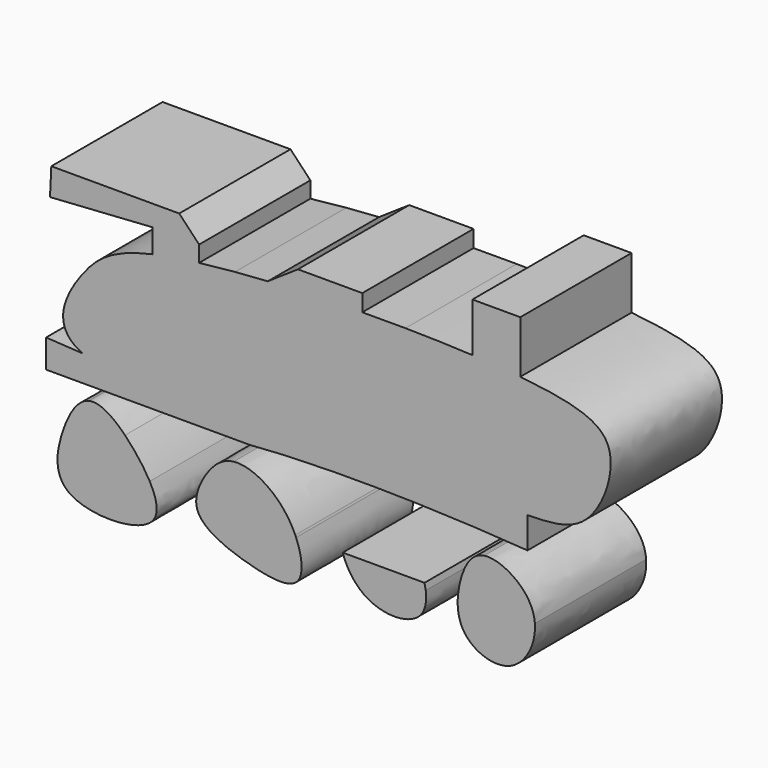
from build123d import *

# Parameters (mm, degrees)
F1_DEPTH = 25.4


with BuildPart() as f1:
    # F0 (on Front) → F1 (new body)
    with BuildSketch(Plane.XZ):
        with BuildLine():
            add(Edge.make_bspline(
                [(0, 6.2092236012), (0.399712228, 6.2271987583), (0.8012564022, 6.2442227103), (1.204486331, 6.2603151334)],
                knots=[0.5892572468, 0.5892572468, 0.5892572468, 0.5892572468, 0.5931096409, 0.5931096409, 0.5931096409, 0.5931096409], degree=3))
            add(Edge.make_bspline(
                [(1.204486331, 6.2603151334), (8.6074057831, 6.5557567752), (16.5785169504, 6.5372221525), (24.2131851795, 6.3264688191)],
                knots=[0.5931096409, 0.5931096409, 0.5931096409, 0.5931096409, 0.6638359458, 0.6638359458, 0.6638359458, 0.6638359458], degree=3))
            add(Edge.make_bspline(
                [(24.2131851795, 6.3264688191), (31.3805995307, 6.1286139261), (38.2514924404, 5.7613485246), (44.0773665905, 5.3254151655)],
                knots=[0.6638359458, 0.6638359458, 0.6638359458, 0.6638359458, 0.7302336879, 0.7302336879, 0.7302336879, 0.7302336879], degree=3))
            Line((44.0773665905, 5.3254151655), (44.0773665905, 10.5862493981))
            Line((44.0773665905, 10.5862493981), (-6.6354808577, 10.5862493981))
            Line((-6.6354808577, 10.5862493981), (-6.6354808577, 5.8050151421))
            add(Edge.make_bspline(
                [(-6.6354808577, 5.8050151421), (-4.875055728, 5.9437108093), (-3.0555777464, 6.0588505348), (-1.1922870019, 6.1524855288)],
                knots=[0.5672778823, 0.5672778823, 0.5672778823, 0.5672778823, 0.5854087698, 0.5854087698, 0.5854087698, 0.5854087698], degree=3))
            add(Edge.make_bspline(
                [(-1.1922870019, 6.1524855288), (-0.5897237764, 6.2718706989), (-0.1594076167, 6.2963081791), (0, 6.2092236012)],
                knots=[0.9136960461, 0.9136960461, 0.9136960461, 0.9136960461, 0.9595308359, 0.9595308359, 0.9595308359, 0.9595308359], degree=3))
        make_face()
        with BuildLine():
            add(Edge.make_bspline(
                [(-1.1922870019, 6.1524855288), (-0.7967833881, 6.172360569), (-0.3993058054, 6.191266721), (0, 6.2092236012)],
                knots=[0.5854087698, 0.5854087698, 0.5854087698, 0.5854087698, 0.5892572468, 0.5892572468, 0.5892572468, 0.5892572468], degree=3))
            add(Edge.make_bspline(
                [(-1.1922870019, 6.1524855288), (-0.5897237764, 6.2718706989), (-0.1594076167, 6.2963081791), (0, 6.2092236012)],
                knots=[0.9136960461, 0.9136960461, 0.9136960461, 0.9136960461, 0.9595308359, 0.9595308359, 0.9595308359, 0.9595308359], degree=3))
        make_face()
        with BuildLine():
            Line((-6.6354808577, 10.5862493981), (44.0773665905, 10.5862493981))
            Line((44.0773665905, 10.5862493981), (44.0773665905, 11.0193416477))
            add(Edge.make_bspline(
                [(42.7648406655, 32.815128364), (44.8295052016, 32.6085821778), (54.6822830844, 31.3655556574), (61.7602511034, 27.526332345), (55.8924998888, 11.2180255433), (47.9060181569, 11.0837244515), (44.0773665905, 11.0193416477)],
                knots=[0.6661346609, 0.6661346609, 0.6661346609, 0.6661346609, 0.6910717984, 0.7961772676, 0.9022891118, 1, 1, 1, 1], degree=3))
            add(Edge.make_bspline(
                [(34.0162292123, 33.4549068765), (37.1606205037, 33.2940351137), (40.1078698163, 33.0809280549), (42.7648406655, 32.815128364)],
                knots=[0.6340436135, 0.6340436135, 0.6340436135, 0.6340436135, 0.6661346609, 0.6661346609, 0.6661346609, 0.6661346609], degree=3))
            add(Edge.make_bspline(
                [(21.7825102865, 33.8114244437), (26.0413693418, 33.7699485679), (30.1758364775, 33.6513871144), (34.0162292123, 33.4549068765)],
                knots=[0.5948493104, 0.5948493104, 0.5948493104, 0.5948493104, 0.6340436135, 0.6340436135, 0.6340436135, 0.6340436135], degree=3))
            add(Edge.make_bspline(
                [(13.9097691545, 33.8017193911), (16.5545841031, 33.8333593914), (19.1915664693, 33.8366569444), (21.7825102865, 33.8114244437)],
                knots=[0.5710048404, 0.5710048404, 0.5710048404, 0.5710048404, 0.5948493104, 0.5948493104, 0.5948493104, 0.5948493104], degree=3))
            add(Edge.make_bspline(
                [(-3.3457321455, 33.1775619897), (2.1686140885, 33.5229891451), (8.058360875, 33.7317188187), (13.9097691545, 33.8017193911)],
                knots=[0.5182511573, 0.5182511573, 0.5182511573, 0.5182511573, 0.5710048404, 0.5710048404, 0.5710048404, 0.5710048404], degree=3))
            add(Edge.make_bspline(
                [(-9.333324452, 32.734493452), (-7.4038813376, 32.9010999132), (-5.4008780095, 33.0488244822), (-3.3457321455, 33.1775619897)],
                knots=[0.4985903473, 0.4985903473, 0.4985903473, 0.4985903473, 0.5182511573, 0.5182511573, 0.5182511573, 0.5182511573], degree=3))
            add(Edge.make_bspline(
                [(-15.8928215503, 32.0572180032), (-13.8354654472, 32.3097697763), (-11.6368180938, 32.5355879122), (-9.333324452, 32.734493452)],
                knots=[0.4751180042, 0.4751180042, 0.4751180042, 0.4751180042, 0.4985903473, 0.4985903473, 0.4985903473, 0.4985903473], degree=3))
            add(Edge.make_bspline(
                [(-19.5242251205, 31.5602992608), (-18.373006051, 31.7360479999), (-17.1597016187, 31.9017015094), (-15.8928215503, 32.0572180032)],
                knots=[0.4606641896, 0.4606641896, 0.4606641896, 0.4606641896, 0.4751180042, 0.4751180042, 0.4751180042, 0.4751180042], degree=3))
            add(Edge.make_bspline(
                [(-24.4341921061, 30.662516132), (-22.9708218581, 30.986326574), (-21.3233394805, 31.2856407804), (-19.5242251205, 31.5602992608)],
                knots=[0.4380759038, 0.4380759038, 0.4380759038, 0.4380759038, 0.4606641896, 0.4606641896, 0.4606641896, 0.4606641896], degree=3))
            add(Edge.make_bspline(
                [(-37.1303893626, 10.5862493981), (-39.6437434771, 11.654431227), (-42.1487635772, 15.6052377938), (-36.5862269371, 25.0979771624), (-31.6870538917, 29.0576233278), (-24.4341921061, 30.662516132)],
                knots=[0.1637001806, 0.1637001806, 0.1637001806, 0.1637001806, 0.2371830276, 0.326122203, 0.4380759038, 0.4380759038, 0.4380759038, 0.4380759038], degree=3))
            add(Edge.make_bspline(
                [(-6.6354808577, 10.5862493981), (-19.0833938627, 9.3964373169), (-31.5313068676, 8.2066252357), (-37.1303893626, 10.5862493981)],
                knots=[0, 0, 0, 0, 0.1637001806, 0.1637001806, 0.1637001806, 0.1637001806], degree=3))
        make_face()
        with BuildLine():
            Line((-43.8378155231, 5.8050151421), (-6.6354808577, 5.8050151421))
            Line((-6.6354808577, 5.8050151421), (-6.6354808577, 10.5862493981))
            add(Edge.make_bspline(
                [(-6.6354808577, 10.5862493981), (-19.0833938627, 9.3964373169), (-31.5313068676, 8.2066252357), (-37.1303893626, 10.5862493981)],
                knots=[0, 0, 0, 0, 0.1637001806, 0.1637001806, 0.1637001806, 0.1637001806], degree=3))
            Line((-37.1303893626, 10.5862493981), (-43.8378155231, 10.9774294734))
            Line((-43.8378155231, 10.9774294734), (-43.8378155231, 5.8050151421))
        make_face()
        with BuildLine():
            add(Edge.make_bspline(
                [(34.0162292123, 33.4549068765), (37.1606205037, 33.2940351137), (40.1078698163, 33.0809280549), (42.7648406655, 32.815128364)],
                knots=[0.6340436135, 0.6340436135, 0.6340436135, 0.6340436135, 0.6661346609, 0.6661346609, 0.6661346609, 0.6661346609], degree=3))
            Line((42.7648406655, 32.815128364), (42.7648406655, 42.3979010901))
            Line((42.7648406655, 42.3979010901), (34.0162292123, 42.3979010901))
            Line((34.0162292123, 42.3979010901), (34.0162292123, 33.4549068765))
        make_face()
        with BuildLine():
            Line((-24.4412293233, 35.0078692423), (-24.4341921061, 30.662516132))
            add(Edge.make_bspline(
                [(-24.4341921061, 30.662516132), (-22.9708218581, 30.986326574), (-21.3233394805, 31.2856407804), (-19.5242251205, 31.5602992608)],
                knots=[0.4380759038, 0.4380759038, 0.4380759038, 0.4380759038, 0.4606641896, 0.4606641896, 0.4606641896, 0.4606641896], degree=3))
            Line((-19.5242251205, 31.5602992608), (-19.5242251205, 35.0078692423))
            Line((-19.5242251205, 35.0078692423), (-24.4412293233, 35.0078692423))
        make_face()
        with BuildLine():
            Line((-19.5242251205, 35.0078692423), (-19.5242251205, 31.5602992608))
            add(Edge.make_bspline(
                [(-19.5242251205, 31.5602992608), (-18.373006051, 31.7360479999), (-17.1597016187, 31.9017015094), (-15.8928215503, 32.0572180032)],
                knots=[0.4606641896, 0.4606641896, 0.4606641896, 0.4606641896, 0.4751180042, 0.4751180042, 0.4751180042, 0.4751180042], degree=3))
            Line((-15.8928215503, 32.0572180032), (-19.5242251205, 35.0078692423))
        make_face()
        Polygon((-43.1230533546, 33.7766769852), (-24.4412293233, 35.0078692423), (-19.5242251205, 35.0078692423), (-19.5242251205, 38.8179787676), (-42.8835022873, 38.8179787676), align=None)
        Polygon((-19.5242251205, 35.0078692423), (-15.8928215503, 32.0572180032), (-15.8928215503, 35.0078692423), (-19.5242251205, 38.8179787676), align=None)
        with BuildLine():
            add(Edge.make_bspline(
                [(-3.3457321455, 33.1775619897), (2.1686140885, 33.5229891451), (8.058360875, 33.7317188187), (13.9097691545, 33.8017193911)],
                knots=[0.5182511573, 0.5182511573, 0.5182511573, 0.5182511573, 0.5710048404, 0.5710048404, 0.5710048404, 0.5710048404], degree=3))
            Line((13.9097691545, 33.8017193911), (13.9097691545, 36.8908382952))
            Line((13.9097691545, 36.8908382952), (2.1533465492, 36.8908382952))
            Line((2.1533465492, 36.8908382952), (-3.3457321455, 33.1775619897))
        make_face()
    extrude(amount=F1_DEPTH)


with BuildPart() as f1b:
    # F0 (on Front) → F1, piece 2 (new body)
    with BuildSketch(Plane.XZ):
        with BuildLine():
            Line((25.2694209994, -5.9887724929), (17.5658932838, -5.9887724929))
            add(Edge.make_bspline(
                [(25.4952859244, -7.1565716616), (25.2365747849, -7.2668342439), (22.9898528221, -8.0096855033), (19.7126906516, -7.284873235), (17.5658932838, -5.9887724929)],
                knots=[0.4315379211, 0.4315379211, 0.4315379211, 0.4315379211, 0.4525822565, 0.6042424432, 0.6042424432, 0.6042424432, 0.6042424432], degree=3))
            add(Edge.make_bspline(
                [(25.2694209994, -5.9887724929), (25.3683799408, -6.3779086848), (25.44467949, -6.7691034162), (25.4952859245, -7.1565716616)],
                knots=[0.2781240565, 0.2781240565, 0.2781240565, 0.2781240565, 0.3019466619, 0.3019466619, 0.3019466619, 0.3019466619], degree=3))
        make_face()
        with BuildLine():
            add(Edge.make_bspline(
                [(25.4952859244, -7.1565716616), (25.2365747849, -7.2668342439), (22.9898528221, -8.0096855033), (19.7126906516, -7.284873235), (17.5658932838, -5.9887724929)],
                knots=[0.4315379211, 0.4315379211, 0.4315379211, 0.4315379211, 0.4525822565, 0.6042424432, 0.6042424432, 0.6042424432, 0.6042424432], degree=3))
            Line((17.5658932838, -5.9887724929), (10.3357936774, -5.9887724929))
            add(Edge.make_bspline(
                [(25.4952859245, -7.1565716616), (25.6978271847, -8.7073291423), (25.0194715693, -13.546496718), (14.8905738998, -13.9825909441), (11.020140813, -8.170368759), (10.3357936774, -5.9887724929)],
                knots=[0.3019466619, 0.3019466619, 0.3019466619, 0.3019466619, 0.3972914652, 0.6113827255, 0.7457766189, 0.7457766189, 0.7457766189, 0.7457766189], degree=3))
        make_face()
    extrude(amount=F1_DEPTH)


with BuildPart() as f1c:
    # F0 (on Front) → F1, piece 3 (new body)
    with BuildSketch(Plane.XZ):
        with BuildLine():
            add(Edge.make_bspline(
                [(1.8248094407, -6.3349300706), (2.9597559177, -9.0339247999), (3.5739908167, -15.4031273729), (-7.0064012474, -13.8188582963), (-16.0179542148, -10.1339589692), (-16.4666651712, -6.7415678942), (-16.4018577434, -5.9887724929)],
                knots=[0.2377172452, 0.2377172452, 0.2377172452, 0.2377172452, 0.3646787095, 0.5306870794, 0.7145579516, 0.7649915026, 0.7649915026, 0.7649915026, 0.7649915026], degree=3))
            add(Edge.make_bspline(
                [(1.8248094222, -6.3349300807), (-0.9007268791, -7.1607290524), (-4.2811435161, -6.9456693749), (-6.9049853005, -5.9887724929)],
                knots=[0.376906454, 0.376906454, 0.376906454, 0.376906454, 0.5231455471, 0.5231455471, 0.5231455471, 0.5231455471], degree=3))
            Line((-6.9049853005, -5.9887724929), (-16.4018577434, -5.9887724929))
        make_face()
        with BuildLine():
            add(Edge.make_bspline(
                [(1.8248094222, -6.3349300807), (-0.9007268791, -7.1607290524), (-4.2811435161, -6.9456693749), (-6.9049853005, -5.9887724929)],
                knots=[0.376906454, 0.376906454, 0.376906454, 0.376906454, 0.5231455471, 0.5231455471, 0.5231455471, 0.5231455471], degree=3))
            add(Edge.make_bspline(
                [(1.674319654, -5.9887724929), (1.726050419, -6.1039709644), (1.7762259024, -6.219394478), (1.8248094407, -6.3349300706)],
                knots=[0.2322824187, 0.2322824187, 0.2322824187, 0.2322824187, 0.2377172452, 0.2377172452, 0.2377172452, 0.2377172452], degree=3))
            Line((1.674319654, -5.9887724929), (-6.9049853005, -5.9887724929))
        make_face()
        with BuildLine():
            Line((-6.9049853005, -5.9887724929), (1.674319654, -5.9887724929))
            add(Edge.make_bspline(
                [(-9.5820352435, 2.1559579764), (-6.6100790469, 2.4892376879), (-1.5624748522, -0.14893978), (1.225366615, -4.9890056426), (1.674319654, -5.9887724929)],
                knots=[0, 0, 0, 0, 0.1851154792, 0.2322824187, 0.2322824187, 0.2322824187, 0.2322824187], degree=3))
            add(Edge.make_bspline(
                [(-6.9049853005, -5.9887724929), (-8.1964155517, -5.5177968463), (-11.753903644, -3.4288979114), (-11.688056374, 0.1446620748), (-9.5820352435, 2.1559579764)],
                knots=[0.5231455471, 0.5231455471, 0.5231455471, 0.5231455471, 0.5951230534, 0.7542148067, 0.7542148067, 0.7542148067, 0.7542148067], degree=3))
        make_face()
        with BuildLine():
            add(Edge.make_bspline(
                [(-6.9049853005, -5.9887724929), (-8.1964155517, -5.5177968463), (-11.753903644, -3.4288979114), (-11.688056374, 0.1446620748), (-9.5820352435, 2.1559579764)],
                knots=[0.5231455471, 0.5231455471, 0.5231455471, 0.5231455471, 0.5951230534, 0.7542148067, 0.7542148067, 0.7542148067, 0.7542148067], degree=3))
            add(Edge.make_bspline(
                [(-16.4018577434, -5.9887724929), (-16.2855090294, -4.6372796173), (-14.633372914, -0.9404484327), (-11.9013670517, 1.8958645615), (-9.5820352435, 2.1559579764)],
                knots=[0.7649915026, 0.7649915026, 0.7649915026, 0.7649915026, 0.8555348092, 1, 1, 1, 1], degree=3))
            Line((-16.4018577434, -5.9887724929), (-6.9049853005, -5.9887724929))
        make_face()
    extrude(amount=F1_DEPTH)


with BuildPart() as f1d:
    # F0 (on Front) → F1, piece 4 (new body)
    with BuildSketch(Plane.XZ):
        with BuildLine():
            add(Edge.make_bspline(
                [(31.3790095867, -5.9887724929), (31.460207537, -5.1005727631), (32.1510856871, -1.4837650362), (33.832432135, 1.5812085942), (36.1721850932, 1.9164072582)],
                knots=[0.7699987611, 0.7699987611, 0.7699987611, 0.7699987611, 0.8266050096, 1, 1, 1, 1], degree=3))
            Line((31.3790095867, -5.9887724929), (45.4263283693, -5.9887724929))
            add(Edge.make_bspline(
                [(36.1721850932, 1.9164072582), (39.1047558728, 2.3365344363), (44.4858759174, -0.7907380392), (45.3800216326, -5.3342820091), (45.4263283693, -5.9887724929)],
                knots=[0, 0, 0, 0, 0.21732768, 0.2532993311, 0.2532993311, 0.2532993311, 0.2532993311], degree=3))
        make_face()
        with BuildLine():
            Line((45.4263283693, -5.9887724929), (31.3790095867, -5.9887724929))
            add(Edge.make_bspline(
                [(45.4263283693, -5.9887724929), (45.6606976863, -9.3013032075), (41.8610307818, -16.6625135346), (31.9901991515, -13.3943385061), (31.1794393746, -8.1718104629), (31.3790095867, -5.9887724929)],
                knots=[0.2532993311, 0.2532993311, 0.2532993311, 0.2532993311, 0.435360342, 0.630870606, 0.7699987611, 0.7699987611, 0.7699987611, 0.7699987611], degree=3))
        make_face()
    extrude(amount=F1_DEPTH)


with BuildPart() as f1e:
    # F0 (on Front) → F1, piece 5 (new body)
    with BuildSketch(Plane.XZ):
        with BuildLine():
            add(Edge.make_bspline(
                [(-29.4240375783, -0.0482268444), (-28.7866548438, -0.6972554841), (-27.1305837874, -2.5694349987), (-25.6135063871, -4.6919174034), (-24.9042103256, -5.9887724929)],
                knots=[0.1516180446, 0.1516180446, 0.1516180446, 0.1516180446, 0.1947634043, 0.2651810746, 0.2651810746, 0.2651810746, 0.2651810746], degree=3))
            add(Edge.make_bspline(
                [(-30.9675135167, -5.9887724929), (-31.1620139659, -5.5917039847), (-31.8581827043, -3.5804512487), (-31.0987248397, -1.5291915244), (-29.4240375783, -0.0482268444)],
                knots=[0.3807868082, 0.3807868082, 0.3807868082, 0.3807868082, 0.3950349644, 0.4525084749, 0.4525084749, 0.4525084749, 0.4525084749], degree=3))
            Line((-30.9675135167, -5.9887724929), (-24.9042103256, -5.9887724929))
        make_face()
        with BuildLine():
            add(Edge.make_bspline(
                [(-30.9675135167, -5.9887724929), (-31.1620139659, -5.5917039847), (-31.8581827043, -3.5804512487), (-31.0987248397, -1.5291915244), (-29.4240375783, -0.0482268444)],
                knots=[0.3807868082, 0.3807868082, 0.3807868082, 0.3807868082, 0.3950349644, 0.4525084749, 0.4525084749, 0.4525084749, 0.4525084749], degree=3))
            add(Edge.make_bspline(
                [(-35.9326340258, 3.3537128475), (-34.0049934694, 3.7444780005), (-31.6638780796, 2.2325387849), (-29.4240375783, -0.0482268444)],
                knots=[0, 0, 0, 0, 0.1516180446, 0.1516180446, 0.1516180446, 0.1516180446], degree=3))
            add(Edge.make_bspline(
                [(-41.5587956864, -5.9887724929), (-41.4187220468, -5.1948417275), (-40.3354460549, -1.0098015608), (-38.2221686619, 2.8895856794), (-35.9326340258, 3.3537128475)],
                knots=[0.7769564787, 0.7769564787, 0.7769564787, 0.7769564787, 0.8199172748, 1, 1, 1, 1], degree=3))
            Line((-41.5587956864, -5.9887724929), (-30.9675135167, -5.9887724929))
        make_face()
        with BuildLine():
            add(Edge.make_bspline(
                [(-24.9042103256, -5.9887724929), (-23.7602606802, -8.0803348179), (-23.2182253262, -10.12183987), (-24.0246758581, -11.6288233698)],
                knots=[0.2651810746, 0.2651810746, 0.2651810746, 0.2651810746, 0.3787503914, 0.3787503914, 0.3787503914, 0.3787503914], degree=3))
            Line((-24.9042103256, -5.9887724929), (-30.9675135167, -5.9887724929))
            add(Edge.make_bspline(
                [(-24.0246758581, -11.6288233698), (-27.6323017774, -9.8853498872), (-29.9980407608, -7.9679303942), (-30.9675135167, -5.9887724929)],
                knots=[0.3097679529, 0.3097679529, 0.3097679529, 0.3097679529, 0.3807868082, 0.3807868082, 0.3807868082, 0.3807868082], degree=3))
        make_face()
        with BuildLine():
            add(Edge.make_bspline(
                [(-24.0246758581, -11.6288233698), (-27.6323017774, -9.8853498872), (-29.9980407608, -7.9679303942), (-30.9675135167, -5.9887724929)],
                knots=[0.3097679529, 0.3097679529, 0.3097679529, 0.3097679529, 0.3807868082, 0.3807868082, 0.3807868082, 0.3807868082], degree=3))
            Line((-30.9675135167, -5.9887724929), (-41.5587956864, -5.9887724929))
            add(Edge.make_bspline(
                [(-24.0246758581, -11.6288233698), (-24.1352084151, -11.8353713637), (-26.3565850136, -15.0482402194), (-41.2317790283, -15.353626471), (-42.0273466413, -8.6444971466), (-41.5587956864, -5.9887724929)],
                knots=[0.3787503914, 0.3787503914, 0.3787503914, 0.3787503914, 0.3943162649, 0.6332511958, 0.7769564787, 0.7769564787, 0.7769564787, 0.7769564787], degree=3))
        make_face()
    extrude(amount=F1_DEPTH)


solid = Compound([f1.part, f1b.part, f1c.part, f1d.part, f1e.part])
